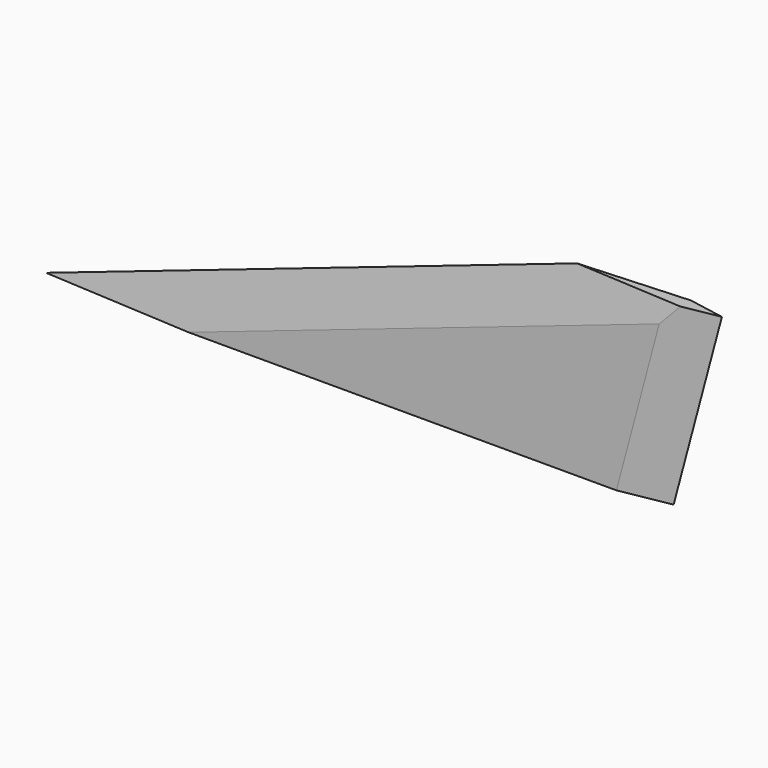
from build123d import *

# Parameters (mm, degrees)
F1_DEPTH = 9.525
F2_SIZE2 = 4.7625
F2_SIZE  = 25.4
F3_SIZE2 = 25.39999
F3_SIZE  = 4.76249
F4_SIZE2 = 4.7625
F4_SIZE  = 25.4
F5_SIZE2 = 25.39999
F5_SIZE  = 4.76249


# Not quite as in the source:
# - a fillet or chamfer is up to 0.001 mm smaller than in the source, because OpenCascade refuses the exact size


with BuildPart() as f1:
    # F0 (on Front) → F1 (new body)
    with BuildSketch(Plane.XZ):
        Polygon((112.3986273699, 65.3573278389), (-167.0013726301, -29.8926721611), (163.1986273699, -29.8926721611), (188.5986273699, 65.3573278389), align=None)
    extrude(amount=F1_DEPTH)

    # F2
    f2_edges = [f1.edges().sort_by_distance(p)[0] for p in [
        (-27.301373, -9.525, 17.732328),
    ]]
    f2_side = f1.faces().sort_by_distance((58.423627, -9.525, 7.810453))[0]
    chamfer(f2_edges, length=F2_SIZE, length2=F2_SIZE2, reference=f2_side)

    # F3 (size 4.7625 and 25.4 in the source; OpenCascade refuses exactly that, so slightly less here)
    f3_edges = [f1.edges().sort_by_distance(p)[0] for p in [
        (-27.301373, 0, 17.732328),
    ]]
    f3_side = f1.faces().sort_by_distance((-27.301373, -2.38125, 17.732328))[0]
    chamfer(f3_edges, length=F3_SIZE, length2=F3_SIZE2, reference=f3_side)

    # F4
    f4_edges = [f1.edges().sort_by_distance(p)[0] for p in [
        (175.772766, -9.525, 17.260346),
    ]]
    f4_side = f1.faces().sort_by_distance((87.753798, -9.525, 1.542673))[0]
    chamfer(f4_edges, length=F4_SIZE, length2=F4_SIZE2, reference=f4_side)

    # F5 (size 4.7625 and 25.4 in the source; OpenCascade refuses exactly that, so slightly less here)
    f5_edges = [f1.edges().sort_by_distance(p)[0] for p in [
        (175.772767, 0, 17.260352),
    ]]
    f5_side = f1.faces().sort_by_distance((175.896628, -2.381619, 17.72483))[0]
    chamfer(f5_edges, length=F5_SIZE, length2=F5_SIZE2, reference=f5_side)


solid = f1.part
